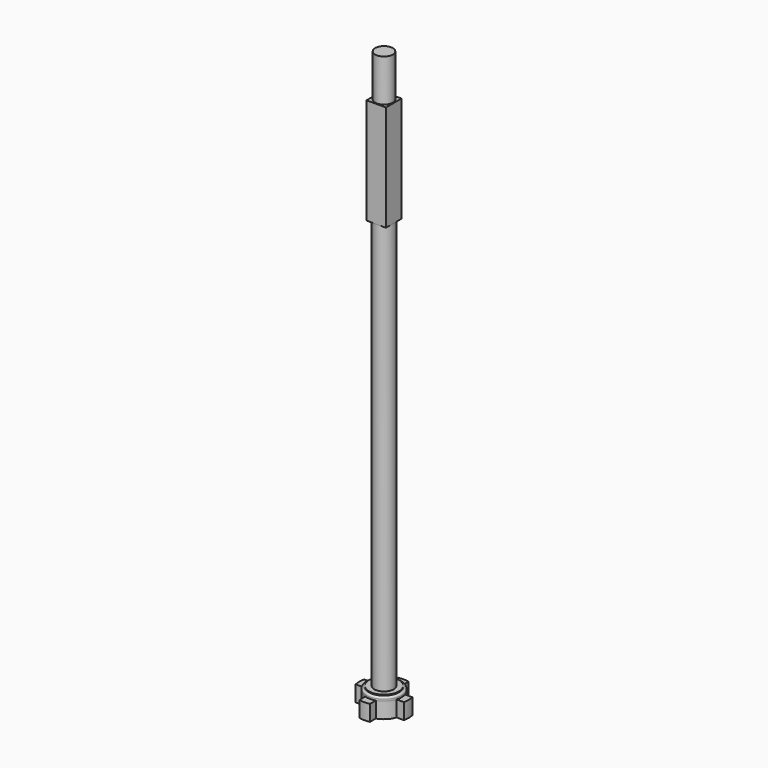
from build123d import *

# Parameters (mm, degrees)
F3_DEPTH        = 34.925
F0_W            = 31.75
F0_H            = 152.4
F7_DEPTH        = 57.15
F7_COPIES_COUNT = 4


# Not quite as in the source:
# - a feature of the source that left no trace in its solid (it failed there, or was rolled back) is left out
# - a pattern or mirror of a feature is missing from the dataset's text; its kind, count and spacing are read off the source's solid


with BuildPart() as f1:
    # F0 (on Front) → F1 (revolve)
    with BuildSketch(Plane.XZ):
        with BuildLine():
            Line((34.925, 73.025), (34.925, 0))
            Line((34.925, 0), (88.9, 0))
            Line((88.9, 0), (88.9, 57.15))
            Line((88.9, 57.15), (63.5, 57.15))
            Line((63.5, 57.15), (63.5, 63.5))
            ThreePointArc((63.5, 63.5), (61.6401280605, 67.9901280605), (57.15, 69.85))
            Line((57.15, 69.85), (54.075, 69.85))
            Line((54.075, 69.85), (54.075, 73.025))
            Line((54.075, 73.025), (34.925, 73.025))
        make_face()
    revolve(axis=Axis((0, 0, -7.5624885379), (0, 0, -1)))

    # F0 (on Front) → F2 (revolve)
    with BuildSketch(Plane.XZ):
        Polygon((0, 1549.4), (0, 0), (34.925, 0), (34.925, 73.025), (34.925, 1549.4), align=None)
    revolve(axis=Axis((0, 0, -7.5624885379), (0, 0, -1)))

    # F0 (on Front) → F3 (join, symmetric)
    with BuildSketch(Plane.XZ):
        Polygon((-34.925, 1549.4), (0, 1549.4), (34.925, 1549.4), (34.925, 1930.4), (31.75, 1930.4), (0, 1930.4), (-34.925, 1930.4), align=None)
    extrude(amount=F3_DEPTH, both=True)

    # F0 (on Front) → F4 (revolve)
    with BuildSketch(Plane.XZ):
        with Locations((15.875, 2006.6)):
            Rectangle(F0_W, F0_H)
    revolve(axis=Axis((0, 0, -7.5624885379), (0, 0, -1)))

    # F6 (on face) → F7 (cut, through all)
    with BuildSketch(Plane(origin=(0, 0, 0), x_dir=(1, 0, 0), z_dir=(0, 0, -1))):
        with BuildLine():
            ThreePointArc((19.05, 60.57513929), (44.9012806053, 44.9012806053), (60.57513929, 19.05))
            Line((60.57513929, 19.05), (86.834944003, 19.05))
            ThreePointArc((86.834944003, 19.05), (62.8617928475, 62.8617928475), (19.05, 86.834944003))
            Line((19.05, 86.834944003), (19.05, 60.57513929))
        make_face()
    f7 = extrude(amount=-F7_DEPTH, mode=Mode.SUBTRACT)

    # F7_copies: F7 ×4 about axis
    f7_copies_axis = Axis((0, 0, 0), (0, 0, 1))
    for i in range(1, F7_COPIES_COUNT):
        add(f7.rotate(f7_copies_axis, i * 360 / F7_COPIES_COUNT), mode=Mode.SUBTRACT)


solid = f1.part
